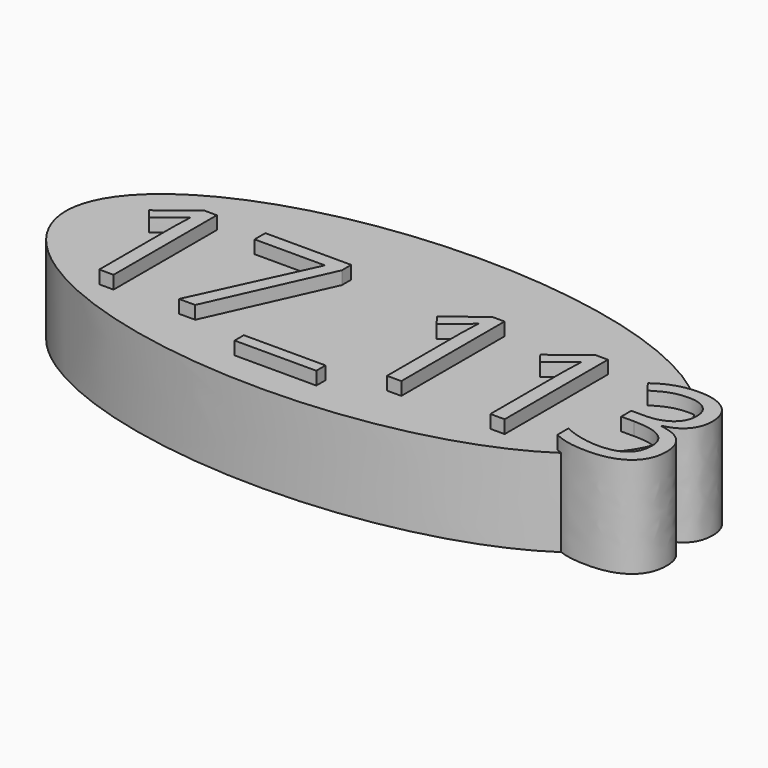
from build123d import *

# Parameters (mm, degrees)
F1_DEPTH     = 22.098
F2_TEXT_SIZE = 45.7160239522
F3_DEPTH     = 25.4


# Not quite as in the source:
# - Text() gives the source's letters only with a copy of the font that has no kerning and outlines rounded to 1/6400 em; it was checked with that copy


with BuildPart() as f1:
    # F0 (on Top) → F1 (new body)
    with BuildSketch(Plane.XY):
        with BuildLine():
            add(Edge.make_bspline(
                [(-77.0800039172, 0), (-77.0800039172, -60.9981022285), (38.5400019586, -30.4990511142), (154.1600078344, 0), (38.5400019586, 30.4990511142), (-77.0800039172, 60.9981022285), (-77.0800039172, 0)],
                knots=[0, 0, 0, 2.0943951024, 2.0943951024, 4.1887902048, 4.1887902048, 6.2831853072, 6.2831853072, 6.2831853072], degree=2, weights=[1, 0.5, 1, 0.5, 1, 0.5, 1]))
        make_face()
    extrude(amount=F1_DEPTH)

    # F2 (on Top) → F3 (join)
    with BuildSketch(Plane.XY):
        with Locations((-64.6710470319, -20.3584531555)):
            Text('17_113', F2_TEXT_SIZE, font='Open Sans', text_align=(TextAlign.LEFT, TextAlign.BOTTOM))
    extrude(amount=F3_DEPTH)


solid = f1.part
